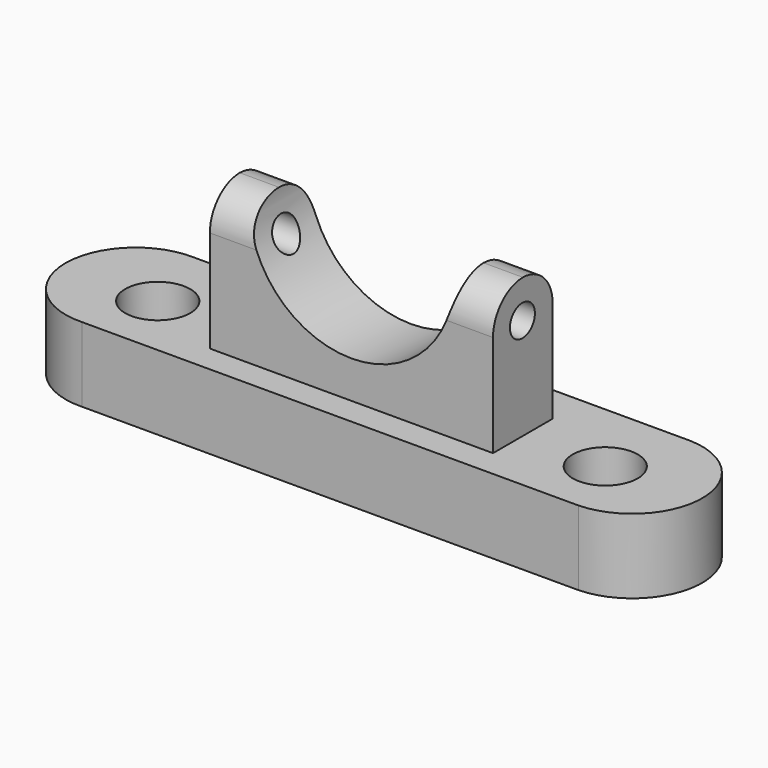
from build123d import *

# Parameters (mm, degrees)
F1_DEPTH    = 25.4
F2_R        = 11.0950895879
F2_R_2      = 11.0767516797
F3_DEPTH    = 51.816
F5_DEPTH    = 12.7
F6_T1_DEPTH = 77.7777149491
F6_T3_DEPTH = 77.7777149491
F7_R        = 5.3247390171
F8_DEPTH    = 189.484


# Not quite as in the source:
# - a fillet or chamfer that OpenCascade refuses, or shapes differently, is made with other operations: its cross-section is extruded or revolved along the edge and cut away or added


with BuildPart() as f1:
    # F0 (on Top) → F1 (new body)
    with BuildSketch(Plane.XY):
        with BuildLine():
            Line((-84.3394622207, -22.0487453043), (-84.3394622207, 25.6632901728))
            ThreePointArc((-84.3394622207, 25.6632901728), (-109.0315538503, 1.8072724342), (-84.3394622207, -22.0487453043))
        make_face()
        Polygon((83.375572493, 25.6632901728), (-84.3394622207, 25.6632901728), (-84.3394622207, -22.0487453043), (83.375572493, -22.0487453043), (84.8214030266, -22.0487453043), (84.8214030266, 25.6632901728), align=None)
        with BuildLine():
            ThreePointArc((84.8214030266, -22.0487453043), (107.965456332, 1.8072724342), (84.8214030266, 25.6632901728))
            Line((84.8214030266, 25.6632901728), (84.8214030266, -22.0487453043))
        make_face()
    extrude(amount=F1_DEPTH)

    # F2 (on face) → F3 (cut)
    with BuildSketch(Plane.XY.offset(25.4)):
        with Locations((-76.1863589287, 0)):
            Circle(F2_R)
        with Locations((76.3475745916, 0)):
            Circle(F2_R_2)
    extrude(amount=-F3_DEPTH, mode=Mode.SUBTRACT)

    # F4 (on Front) → F5 (join, symmetric)
    with BuildSketch(Plane.XZ):
        with BuildLine():
            Line((-34.8596895088, 72.9802176356), (-48.2503287494, 72.9802176356))
            Line((-48.2503287494, 72.9802176356), (-48.2503287494, 0))
            Line((-48.2503287494, 0), (48.2503287494, 0))
            Line((48.2503287494, 0), (48.2503287494, 72.9802176356))
            Line((48.2503287494, 72.9802176356), (34.8596895088, 72.9802176356))
            ThreePointArc((34.8596895088, 72.9802176356), (0, 38.1205281268), (-34.8596895088, 72.9802176356))
        make_face()
    extrude(amount=F5_DEPTH, both=True)

    # F6: fillet of radius 12.8774151417 on 4 edges, made by hand

    # F6_s2 → F6_t1 (cut)
    with BuildSketch(Plane.YZ.offset(-80.4438666037)):
        with BuildLine():
            ThreePointArc((-12.7, 60.1028024939), (-8.9282924292, 69.2085100648), (0.1774151417, 72.9802176356))
            Line((0.1774151417, 72.9802176356), (-12.7, 72.9802176356))
            Line((-12.7, 72.9802176356), (-12.7, 60.1028024939))
        make_face()
        with BuildLine():
            ThreePointArc((12.7, 60.1028024939), (8.9282924292, 69.2085100648), (-0.1774151417, 72.9802176356))
            Line((-0.1774151417, 72.9802176356), (12.7, 72.9802176356))
            Line((12.7, 72.9802176356), (12.7, 60.1028024939))
        make_face()
    extrude(amount=F6_T1_DEPTH, mode=Mode.SUBTRACT)

    # F6_s4 → F6_t3 (cut)
    with BuildSketch(Plane.YZ.offset(2.6661516546)):
        with BuildLine():
            ThreePointArc((12.7, 60.1028024939), (8.9282924292, 69.2085100648), (-0.1774151417, 72.9802176356))
            Line((-0.1774151417, 72.9802176356), (12.7, 72.9802176356))
            Line((12.7, 72.9802176356), (12.7, 60.1028024939))
        make_face()
        with BuildLine():
            ThreePointArc((-12.7, 60.1028024939), (-8.9282924292, 69.2085100648), (0.1774151417, 72.9802176356))
            Line((0.1774151417, 72.9802176356), (-12.7, 72.9802176356))
            Line((-12.7, 72.9802176356), (-12.7, 60.1028024939))
        make_face()
    extrude(amount=F6_T3_DEPTH, mode=Mode.SUBTRACT)

    # F7 (on face) → F8 (cut)
    with BuildSketch(Plane(origin=(-48.2503287494, 0, 0), x_dir=(0, -1, 0), z_dir=(-1, 0, 0))):
        with Locations((0.1774151417, 60.1028024939)):
            Circle(F7_R)
    extrude(amount=-F8_DEPTH, mode=Mode.SUBTRACT)


solid = f1.part
